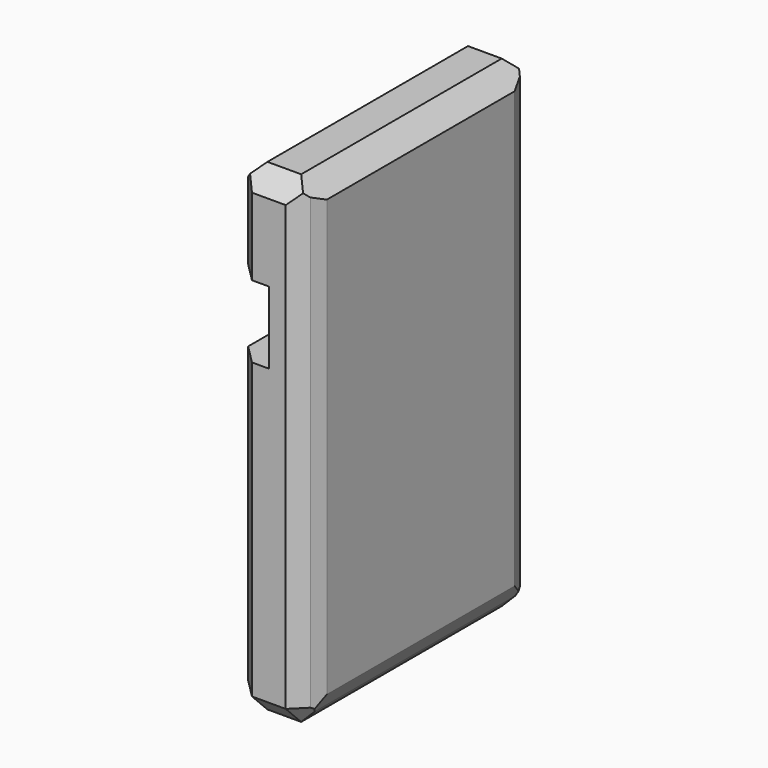
from build123d import *

# Parameters (mm, degrees)
F1_DEPTH    = 76.2
F2_SIZE     = 5.08
F3_SIZE     = 5.08
F4_SIZE     = 5.08
F5_T1_DEPTH = 92.1682991577
F5_T3_DEPTH = 133.3862799398
F5_T5_DEPTH = 77.5062799398


# Not quite as in the source:
# - a fillet or chamfer that OpenCascade refuses, or shapes differently, is made with other operations: its cross-section is extruded or revolved along the edge and cut away or added


with BuildPart() as f1:
    # F0 (on Front) → F1 (new body)
    with BuildSketch(Plane.XZ):
        Polygon((-5.919593852, -19.1378965259), (13.130406148, -19.1378965259), (13.130406148, 107.8621034741), (-5.919593852, 107.8621034741), (-5.919593852, 82.4621034741), (3.605406148, 82.4621034741), (3.605406148, 63.4121034741), (-5.919593852, 63.4121034741), align=None)
    extrude(amount=F1_DEPTH)

    # F2
    f2_edges = [f1.edges().sort_by_distance(p)[0] for p in [
        (-5.919594, 0, 95.162103),
        (13.130406, 0, 44.362103),
        (3.605406, 0, -19.137897),
        (-5.919594, 0, 22.137103),
        (-5.919594, -38.1, -19.137897),
        (-5.919594, -76.2, 22.137103),
        (13.130406, -38.1, -19.137897),
        (3.605406, -76.2, -19.137897),
        (13.130406, -76.2, 44.362103),
        (3.605406, -76.2, 107.862103),
        (-5.919594, -38.1, 107.862103),
    ]]
    chamfer(f2_edges, length=F2_SIZE)

    # F3
    f3_edges = [f1.edges().sort_by_distance(p)[0] for p in [
        (-5.919594, -76.2, 92.622103),
    ]]
    chamfer(f3_edges, length=F3_SIZE)

    # F4
    f4_edges = [f1.edges().sort_by_distance(p)[0] for p in [
        (3.605406, 0, 107.862103),
    ]]
    chamfer(f4_edges, length=F4_SIZE)

    # F5: chamfer of 5.08 on 4 edges, made by hand

    # F5_s2 → F5_t1 (cut)
    with BuildSketch(Plane.XZ.offset(-7.9841495789)):
        Polygon((8.050406148, 107.8621034741), (13.130406148, 102.7821034741), (13.130406148, 107.8621034741), align=None)
    extrude(amount=F5_T1_DEPTH, mode=Mode.SUBTRACT)

    # F5_s4 → F5_t3 (cut)
    with BuildSketch(Plane.XY.offset(-19.7910364957)):
        Polygon((13.130406148, -69.0157951031), (11.6425085964, -72.6078975516), (13.130406148, -71.12), align=None)
        Polygon((11.6425085964, -3.5921024484), (13.130406148, -7.1842048969), (13.130406148, -5.08), align=None)
    extrude(amount=F5_T3_DEPTH, mode=Mode.SUBTRACT)

    # F5_s6 → F5_t5 (cut)
    with BuildSketch(Plane.XZ.offset(-0.6531399699)):
        Polygon((13.130406148, -11.953691629), (11.6425085964, -15.5457940774), (13.130406148, -14.0578965259), align=None)
    extrude(amount=F5_T5_DEPTH, mode=Mode.SUBTRACT)


solid = f1.part
